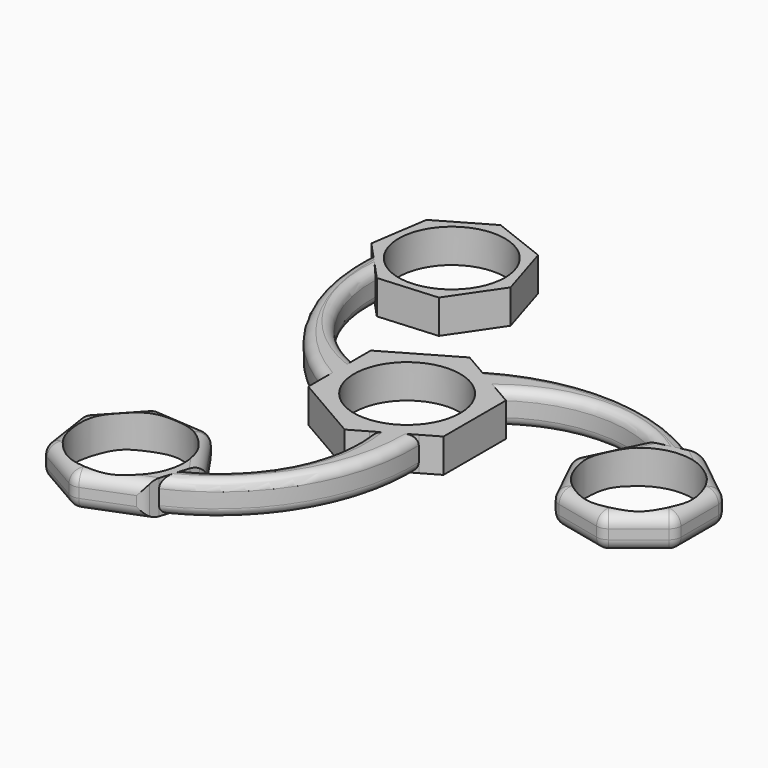
from build123d import *

# Parameters (mm, degrees)
F0_R          = 11
F1_DEPTH      = 7
F2_T4_ANGLE   = 80.8071756388
F2_T10_ANGLE  = 80.8071756388
F2_T16_ANGLE  = 89.7153399134
F2_T22_ANGLE  = 89.7153399134
F2_T28_ANGLE  = 80.8071756388
F2_T34_ANGLE  = 89.7153399134
F2_T40_ANGLE  = 80.8071756388
F2_T46_ANGLE  = 89.7153399134
F2_T52_ANGLE  = 89.7153399134
F2_T58_ANGLE  = 80.8071756388
F2_T64_ANGLE  = 89.7153399134
F2_T70_ANGLE  = 80.8071756388
F3_T1_DEPTH   = 9.7342520499
F3_T3_DEPTH   = 9.7342520499
F3_T5_DEPTH   = 9.7342520499
F3_T7_DEPTH   = 9.7342520499
F3_T9_DEPTH   = 17.188188597
F3_T11_DEPTH  = 2
F3_T13_DEPTH  = 13.0196827351
F3_T15_DEPTH  = 17.188188597
F3_T17_DEPTH  = 9.7342520499
F3_T19_DEPTH  = 9.7342520499
F3_T21_DEPTH  = 9.7342520499
F3_T23_DEPTH  = 9.7342520499
F3_T28_DEPTH  = 2.55
F3_T34_DEPTH  = 2.55
F3_T40_DEPTH  = 2.55
F3_T46_DEPTH  = 2.55
F3_T52_DEPTH  = 2.55
F3_T58_DEPTH  = 2.55
F3_T64_DEPTH  = 2.55
F3_T70_DEPTH  = 2.55
F3_T76_DEPTH  = 2.55
F3_T82_DEPTH  = 2.55
F3_T88_DEPTH  = 2.55
F3_T94_DEPTH  = 2.55
F3_T100_DEPTH = 2.55
F3_T106_DEPTH = 2.55
F3_T112_DEPTH = 2.55
F3_T118_DEPTH = 2.55
F3_T124_DEPTH = 2.55
F3_T130_DEPTH = 2.55
F3_T136_DEPTH = 2.55
F3_T142_DEPTH = 2.55
F3_T148_DEPTH = 17.188188597
F3_T153_DEPTH = 17.188188597
F3_T158_DEPTH = 17.188188597
F3_T163_DEPTH = 17.188188597


# Not quite as in the source:
# - a fillet or chamfer that OpenCascade refuses, or shapes differently, is made with other operations: its cross-section is extruded or revolved along the edge and cut away or added


with BuildPart() as f1:
    # F0 (on Top) → F1 (new body)
    with BuildSketch(Plane.XY):
        with BuildLine():
            Line((60.599063076, -6.071062572), (60.599063076, 6.071062572))
            Line((60.599063076, 6.071062572), (51.1059673744, 13.6415537722))
            Line((51.1059673744, 13.6415537722), (48.1465431954, 12.9660845153))
            ThreePointArc((48.1465431954, 12.9660845153), (25.9998304631, 20.2415563694), (3.5, 14.1450815951))
            Line((3.5, 14.1450815951), (0, 16.1658075373))
            Line((0, 16.1658075373), (-14, 8.0829037687))
            Line((-14, 8.0829037687), (-14, 4.0414518843))
            ThreePointArc((-14, 4.0414518843), (-26.7485538416, 14.727206882), (-31.1728589248, 30.7626834715))
            Line((-31.1728589248, 30.7626834715), (-29.1081732994, 28.5374815803))
            Line((-29.1081732994, 28.5374815803), (-17, 29.4448637287))
            Line((-17, 29.4448637287), (-10.1600973589, 39.4771583252))
            Line((-10.1600973589, 39.4771583252), (-13.7390515734, 51.0798429173))
            Line((-13.7390515734, 51.0798429173), (-25.0418371227, 55.5158593554))
            Line((-25.0418371227, 55.5158593554), (-35.5572259533, 49.4447967834))
            Line((-35.5572259533, 49.4447967834), (-37.366915801, 37.4382891451))
            Line((-37.366915801, 37.4382891451), (-35.3022301756, 35.2130872539))
            ThreePointArc((-35.3022301756, 35.2130872539), (-30.5296172596, 12.3957354905), (-14, -4.0414518843))
            Line((-14, -4.0414518843), (-14, -8.0829037687))
            Line((-14, -8.0829037687), (0, -16.1658075373))
            Line((0, -16.1658075373), (3.5, -14.1450815951))
            ThreePointArc((3.5, -14.1450815951), (0.6201416342, -30.5285305823), (-11.0548359125, -42.3778294732))
            Line((-11.0548359125, -42.3778294732), (-10.1600973589, -39.4771583252))
            Line((-10.1600973589, -39.4771583252), (-17, -29.4448637287))
            Line((-17, -29.4448637287), (-29.1081732994, -28.5374815803))
            Line((-29.1081732994, -28.5374815803), (-37.366915801, -37.4382891451))
            Line((-37.366915801, -37.4382891451), (-35.5572259533, -49.4447967834))
            Line((-35.5572259533, -49.4447967834), (-25.0418371227, -55.5158593554))
            Line((-25.0418371227, -55.5158593554), (-13.7390515734, -51.0798429173))
            Line((-13.7390515734, -51.0798429173), (-12.8443130198, -48.1791717693))
            ThreePointArc((-12.8443130198, -48.1791717693), (4.5297867965, -32.6372918599), (10.5, -10.1036297108))
            Line((10.5, -10.1036297108), (14, -8.0829037687))
            Line((14, -8.0829037687), (14, 0))
            Line((14, 0), (14, 8.0829037687))
            Line((14, 8.0829037687), (10.5, 10.1036297108))
            ThreePointArc((10.5, 10.1036297108), (26.1284122074, 15.8013237004), (42.2276948373, 11.6151460017))
            Line((42.2276948373, 11.6151460017), (39.2682706583, 10.9396767449))
            Line((39.2682706583, 10.9396767449), (34, 0))
            Line((34, 0), (39.2682706583, -10.9396767449))
            Line((39.2682706583, -10.9396767449), (51.1059673744, -13.6415537722))
            Line((51.1059673744, -13.6415537722), (60.599063076, -6.071062572))
        make_face()
        with Locations((-23.9961858727, -41.5626131193)):
            Circle(F0_R, mode=Mode.SUBTRACT)
        Circle(F0_R, mode=Mode.SUBTRACT)
        with Locations((47.9923717453, 0)):
            Circle(F0_R, mode=Mode.SUBTRACT)
        with Locations((-23.9961858727, 41.5626131193)):
            Circle(F0_R, mode=Mode.SUBTRACT)
    extrude(amount=F1_DEPTH)

    # F2: fillet of radius 2 on 12 edges, made by hand


with BuildPart() as f2_tool2:
    # F2_s3 → F2_t4 (revolve)
    with BuildSketch(Plane(origin=(6.6396058585, 31.4629160647, 0), x_dir=(0, 0, 1), z_dir=(0.2064819747, 0.9784504045, 0))):
        with BuildLine():
            ThreePointArc((7.0004, -40.1191282619), (6.4142135624, -41.5343075097), (4.9990343146, -42.1204939473))
            Line((4.9990343146, -42.1204939473), (4.9990343146, -42.3206305158))
            ThreePointArc((4.9990343146, -42.3206305158), (5.9995171573, -42.3202305158), (7, -42.3202305158))
            Line((7, -42.3202305158), (7.2001365685, -42.1200939473))
            ThreePointArc((7.2001365685, -42.1200939473), (7.2001365685, -41.1196111046), (7.2005365685, -40.1191282619))
            Line((7.2005365685, -40.1191282619), (7.0004, -40.1191282619))
        make_face()
    revolve(axis=Axis((5.1756088553, 31.7718627325, 7), (0, 0, 1)), revolution_arc=F2_T4_ANGLE)

    split(bisect_by=Plane.YZ.offset(-14), keep=Keep.BOTTOM)

    split(bisect_by=Plane(origin=(-1.4128724102, -1.310954016, 0), x_dir=(0, 0, 1), z_dir=(-0.7330518718, -0.6801727378, 0)), keep=Keep.TOP)


with BuildPart() as f1_1:
    add(f1.part)

    # F2_t1: cut F2_tool2
    add(f2_tool2.part, mode=Mode.SUBTRACT)


with BuildPart() as f2_tool8:
    # F2_s9 → F2_t10 (revolve)
    with BuildSketch(Plane(origin=(-30.5674875184, -9.9813906878, 0), x_dir=(0, 0, 1), z_dir=(-0.950603894, -0.3104065668, 0))):
        with BuildLine():
            ThreePointArc((7.0004, -40.1191282619), (6.4142135624, -41.5343075097), (4.9990343146, -42.1204939473))
            Line((4.9990343146, -42.1204939473), (4.9990343146, -42.3206305158))
            ThreePointArc((4.9990343146, -42.3206305158), (5.9995171573, -42.3202305158), (7, -42.3202305158))
            Line((7, -42.3202305158), (7.2001365685, -42.1200939473))
            ThreePointArc((7.2001365685, -42.1200939473), (7.2001365685, -41.1196111046), (7.2005365685, -40.1191282619))
            Line((7.2005365685, -40.1191282619), (7.0004, -40.1191282619))
        make_face()
    revolve(axis=Axis((-30.1030446796, -11.4037226175, 7), (0, 0, 1)), revolution_arc=F2_T10_ANGLE)

    split(bisect_by=Plane(origin=(7, -12.124355653, 0), x_dir=(0, 0, 1), z_dir=(0.5, -0.8660254038, 0)), keep=Keep.TOP)

    split(bisect_by=Plane(origin=(1.8417556862, -0.5681063915, 0), x_dir=(0, 0, 1), z_dir=(0.9555728058, -0.2947551744, 0)), keep=Keep.TOP)


with BuildPart() as f1_2:
    add(f1_1.part)

    # F2_t7: cut F2_tool8
    add(f2_tool8.part, mode=Mode.SUBTRACT)


with BuildPart() as f2_tool14:
    # F2_s15 → F2_t16 (revolve)
    with BuildSketch(Plane(origin=(2.8896760525, -9.1175868054, 0), x_dir=(0, 0, 1), z_dir=(-0.3021235761, 0.9532687684, 0))):
        with BuildLine():
            ThreePointArc((7.0004, 1.5102904536), (6.4142135624, 0.0951112058), (4.9990343146, -0.4910752318))
            Line((4.9990343146, -0.4910752318), (4.9990343146, -0.6912118004))
            ThreePointArc((4.9990343146, -0.6912118004), (5.9995171573, -0.6908118004), (7, -0.6908118004))
            Line((7, -0.6908118004), (7.2001365685, -0.4906752318))
            ThreePointArc((7.2001365685, -0.4906752318), (7.2001365685, 0.5098076109), (7.2005365685, 1.5102904536))
            Line((7.2005365685, 1.5102904536), (7.0004, 1.5102904536))
        make_face()
    revolve(axis=Axis((-24.2357516221, -17.714565418, 7), (0, 0, -1)), revolution_arc=F2_T16_ANGLE)

    split(bisect_by=Plane(origin=(1.8417556862, -0.5681063915, 0), x_dir=(0, 0, 1), z_dir=(0.9555728058, -0.2947551744, 0)), keep=Keep.TOP)

    split(bisect_by=Plane(origin=(7, -12.124355653, 0), x_dir=(0, 0, 1), z_dir=(0.5, -0.8660254038, 0)), keep=Keep.TOP)


with BuildPart() as f1_3:
    add(f1_2.part)

    # F2_t13: cut F2_tool14
    add(f2_tool14.part, mode=Mode.SUBTRACT)


with BuildPart() as f2_tool20:
    # F2_s21 → F2_t22 (revolve)
    with BuildSketch(Plane(origin=(6.4512237685, 7.0613262729, 0), x_dir=(0, 0, 1), z_dir=(-0.674493182, -0.7382810762, 0))):
        with BuildLine():
            ThreePointArc((7.0004, 1.5102904536), (6.4142135624, 0.0951112058), (4.9990343146, -0.4910752318))
            Line((4.9990343146, -0.4910752318), (4.9990343146, -0.6912118004))
            ThreePointArc((4.9990343146, -0.6912118004), (5.9995171573, -0.6908118004), (7, -0.6908118004))
            Line((7, -0.6908118004), (7.2001365685, -0.4906752318))
            ThreePointArc((7.2001365685, -0.4906752318), (7.2001365685, 0.5098076109), (7.2005365685, 1.5102904536))
            Line((7.2005365685, 1.5102904536), (7.0004, 1.5102904536))
        make_face()
    revolve(axis=Axis((27.45913948, -12.1314938756, 7), (0, 0, -1)), revolution_arc=F2_T22_ANGLE)

    split(bisect_by=Plane(origin=(-0.428883276, 1.8790604075, 0), x_dir=(0, 0, 1), z_dir=(-0.222520934, 0.9749279122, 0)), keep=Keep.TOP)

    split(bisect_by=Plane(origin=(7, 12.124355653, 0), x_dir=(0, 0, 1), z_dir=(0.5, 0.8660254038, 0)), keep=Keep.TOP)


with BuildPart() as f1_4:
    add(f1_3.part)

    # F2_t19: cut F2_tool20
    add(f2_tool20.part, mode=Mode.SUBTRACT)


with BuildPart() as f2_tool26:
    # F2_s27 → F2_t28 (revolve)
    with BuildSketch(Plane(origin=(23.9278816599, -21.4815253769, 0), x_dir=(0, 0, 1), z_dir=(0.7441219193, -0.6680438378, 0))):
        with BuildLine():
            ThreePointArc((7.0004, -40.1191282619), (6.4142135624, -41.5343075097), (4.9990343146, -42.1204939473))
            Line((4.9990343146, -42.1204939473), (4.9990343146, -42.3206305158))
            ThreePointArc((4.9990343146, -42.3206305158), (5.9995171573, -42.3202305158), (7, -42.3202305158))
            Line((7, -42.3202305158), (7.2001365685, -42.1200939473))
            ThreePointArc((7.2001365685, -42.1200939473), (7.2001365685, -41.1196111046), (7.2005365685, -40.1191282619))
            Line((7.2005365685, -40.1191282619), (7.0004, -40.1191282619))
        make_face()
    revolve(axis=Axis((24.9274358243, -20.368140115, 7), (0, 0, 1)), revolution_arc=F2_T28_ANGLE)

    split(bisect_by=Plane(origin=(7, 12.124355653, 0), x_dir=(0, 0, 1), z_dir=(0.5, 0.8660254038, 0)), keep=Keep.TOP)

    split(bisect_by=Plane(origin=(-0.428883276, 1.8790604075, 0), x_dir=(0, 0, 1), z_dir=(-0.222520934, 0.9749279122, 0)), keep=Keep.TOP)


with BuildPart() as f1_5:
    add(f1_4.part)

    # F2_t25: cut F2_tool26
    add(f2_tool26.part, mode=Mode.SUBTRACT)


with BuildPart() as f2_tool32:
    # F2_s33 → F2_t34 (revolve)
    with BuildSketch(Plane(origin=(-9.3408998209, 2.0562605326, 0), x_dir=(0, 0, 1), z_dir=(0.9766167581, -0.2149876922, 0))):
        with BuildLine():
            ThreePointArc((7.0004, 1.5102904536), (6.4142135624, 0.0951112058), (4.9990343146, -0.4910752318))
            Line((4.9990343146, -0.4910752318), (4.9990343146, -0.6912118004))
            ThreePointArc((4.9990343146, -0.6912118004), (5.9995171573, -0.6908118004), (7, -0.6908118004))
            Line((7, -0.6908118004), (7.2001365685, -0.4906752318))
            ThreePointArc((7.2001365685, -0.4906752318), (7.2001365685, 0.5098076109), (7.2005365685, 1.5102904536))
            Line((7.2005365685, 1.5102904536), (7.0004, 1.5102904536))
        make_face()
    revolve(axis=Axis((-3.2233878579, 29.8460592935, 7), (0, 0, -1)), revolution_arc=F2_T34_ANGLE)

    split(bisect_by=Plane(origin=(-1.4128724102, -1.310954016, 0), x_dir=(0, 0, 1), z_dir=(-0.7330518718, -0.6801727378, 0)), keep=Keep.TOP)

    split(bisect_by=Plane.YZ.offset(-14), keep=Keep.BOTTOM)


with BuildPart() as f1_6:
    add(f1_5.part)

    # F2_t31: cut F2_tool32
    add(f2_tool32.part, mode=Mode.SUBTRACT)


with BuildPart() as f2_tool38:
    # F2_s39 → F2_t40 (revolve)
    with BuildSketch(Plane(origin=(-30.5674875184, -9.9813906878, 0), x_dir=(0, 0, 1), z_dir=(-0.950603894, -0.3104065668, 0))):
        with BuildLine():
            ThreePointArc((2.0009656854, -42.1204939473), (0.5857864376, -41.5343075097), (-0.0004, -40.1191282619))
            Line((-0.0004, -40.1191282619), (-0.2005365685, -40.1191282619))
            ThreePointArc((-0.2005365685, -40.1191282619), (-0.2001365685, -41.1196111046), (-0.2001365685, -42.1200939473))
            Line((-0.2001365685, -42.1200939473), (0, -42.3202305158))
            ThreePointArc((0, -42.3202305158), (1.0004828427, -42.3202305158), (2.0009656854, -42.3206305158))
            Line((2.0009656854, -42.3206305158), (2.0009656854, -42.1204939473))
        make_face()
    revolve(axis=Axis((-30.1030446796, -11.4037226175, 0), (0, 0, 1)), revolution_arc=F2_T40_ANGLE)

    split(bisect_by=Plane(origin=(7, -12.124355653, 0), x_dir=(0, 0, 1), z_dir=(0.5, -0.8660254038, 0)), keep=Keep.TOP)

    split(bisect_by=Plane(origin=(1.8417556862, -0.5681063915, 0), x_dir=(0, 0, 1), z_dir=(0.9555728058, -0.2947551744, 0)), keep=Keep.TOP)


with BuildPart() as f1_7:
    add(f1_6.part)

    # F2_t37: cut F2_tool38
    add(f2_tool38.part, mode=Mode.SUBTRACT)


with BuildPart() as f2_tool44:
    # F2_s45 → F2_t46 (revolve)
    with BuildSketch(Plane(origin=(2.8896760525, -9.1175868054, 0), x_dir=(0, 0, 1), z_dir=(-0.3021235761, 0.9532687684, 0))):
        with BuildLine():
            ThreePointArc((2.0009656854, -0.4910752318), (0.5857864376, 0.0951112058), (-0.0004, 1.5102904536))
            Line((-0.0004, 1.5102904536), (-0.2005365685, 1.5102904536))
            ThreePointArc((-0.2005365685, 1.5102904536), (-0.2001365685, 0.5098076109), (-0.2001365685, -0.4906752318))
            Line((-0.2001365685, -0.4906752318), (0, -0.6908118004))
            ThreePointArc((0, -0.6908118004), (1.0004828427, -0.6908118004), (2.0009656854, -0.6912118004))
            Line((2.0009656854, -0.6912118004), (2.0009656854, -0.4910752318))
        make_face()
    revolve(axis=Axis((-24.2357516221, -17.714565418, 0), (0, 0, -1)), revolution_arc=F2_T46_ANGLE)

    split(bisect_by=Plane(origin=(1.8417556862, -0.5681063915, 0), x_dir=(0, 0, 1), z_dir=(0.9555728058, -0.2947551744, 0)), keep=Keep.TOP)

    split(bisect_by=Plane(origin=(7, -12.124355653, 0), x_dir=(0, 0, 1), z_dir=(0.5, -0.8660254038, 0)), keep=Keep.TOP)


with BuildPart() as f1_8:
    add(f1_7.part)

    # F2_t43: cut F2_tool44
    add(f2_tool44.part, mode=Mode.SUBTRACT)


with BuildPart() as f2_tool50:
    # F2_s51 → F2_t52 (revolve)
    with BuildSketch(Plane(origin=(6.4512237685, 7.0613262729, 0), x_dir=(0, 0, 1), z_dir=(-0.674493182, -0.7382810762, 0))):
        with BuildLine():
            ThreePointArc((2.0009656854, -0.4910752318), (0.5857864376, 0.0951112058), (-0.0004, 1.5102904536))
            Line((-0.0004, 1.5102904536), (-0.2005365685, 1.5102904536))
            ThreePointArc((-0.2005365685, 1.5102904536), (-0.2001365685, 0.5098076109), (-0.2001365685, -0.4906752318))
            Line((-0.2001365685, -0.4906752318), (0, -0.6908118004))
            ThreePointArc((0, -0.6908118004), (1.0004828427, -0.6908118004), (2.0009656854, -0.6912118004))
            Line((2.0009656854, -0.6912118004), (2.0009656854, -0.4910752318))
        make_face()
    revolve(axis=Axis((27.45913948, -12.1314938756, 0), (0, 0, -1)), revolution_arc=F2_T52_ANGLE)

    split(bisect_by=Plane(origin=(-0.428883276, 1.8790604075, 0), x_dir=(0, 0, 1), z_dir=(-0.222520934, 0.9749279122, 0)), keep=Keep.TOP)

    split(bisect_by=Plane(origin=(7, 12.124355653, 0), x_dir=(0, 0, 1), z_dir=(0.5, 0.8660254038, 0)), keep=Keep.TOP)


with BuildPart() as f1_9:
    add(f1_8.part)

    # F2_t49: cut F2_tool50
    add(f2_tool50.part, mode=Mode.SUBTRACT)


with BuildPart() as f2_tool56:
    # F2_s57 → F2_t58 (revolve)
    with BuildSketch(Plane(origin=(23.9278816599, -21.4815253769, 0), x_dir=(0, 0, 1), z_dir=(0.7441219193, -0.6680438378, 0))):
        with BuildLine():
            ThreePointArc((2.0009656854, -42.1204939473), (0.5857864376, -41.5343075097), (-0.0004, -40.1191282619))
            Line((-0.0004, -40.1191282619), (-0.2005365685, -40.1191282619))
            ThreePointArc((-0.2005365685, -40.1191282619), (-0.2001365685, -41.1196111046), (-0.2001365685, -42.1200939473))
            Line((-0.2001365685, -42.1200939473), (0, -42.3202305158))
            ThreePointArc((0, -42.3202305158), (1.0004828427, -42.3202305158), (2.0009656854, -42.3206305158))
            Line((2.0009656854, -42.3206305158), (2.0009656854, -42.1204939473))
        make_face()
    revolve(axis=Axis((24.9274358243, -20.368140115, 0), (0, 0, 1)), revolution_arc=F2_T58_ANGLE)

    split(bisect_by=Plane(origin=(7, 12.124355653, 0), x_dir=(0, 0, 1), z_dir=(0.5, 0.8660254038, 0)), keep=Keep.TOP)

    split(bisect_by=Plane(origin=(-0.428883276, 1.8790604075, 0), x_dir=(0, 0, 1), z_dir=(-0.222520934, 0.9749279122, 0)), keep=Keep.TOP)


with BuildPart() as f1_10:
    add(f1_9.part)

    # F2_t55: cut F2_tool56
    add(f2_tool56.part, mode=Mode.SUBTRACT)


with BuildPart() as f2_tool62:
    # F2_s63 → F2_t64 (revolve)
    with BuildSketch(Plane(origin=(-9.3408998209, 2.0562605326, 0), x_dir=(0, 0, 1), z_dir=(0.9766167581, -0.2149876922, 0))):
        with BuildLine():
            ThreePointArc((2.0009656854, -0.4910752318), (0.5857864376, 0.0951112058), (-0.0004, 1.5102904536))
            Line((-0.0004, 1.5102904536), (-0.2005365685, 1.5102904536))
            ThreePointArc((-0.2005365685, 1.5102904536), (-0.2001365685, 0.5098076109), (-0.2001365685, -0.4906752318))
            Line((-0.2001365685, -0.4906752318), (0, -0.6908118004))
            ThreePointArc((0, -0.6908118004), (1.0004828427, -0.6908118004), (2.0009656854, -0.6912118004))
            Line((2.0009656854, -0.6912118004), (2.0009656854, -0.4910752318))
        make_face()
    revolve(axis=Axis((-3.2233878579, 29.8460592935, 0), (0, 0, -1)), revolution_arc=F2_T64_ANGLE)

    split(bisect_by=Plane(origin=(-1.4128724102, -1.310954016, 0), x_dir=(0, 0, 1), z_dir=(-0.7330518718, -0.6801727378, 0)), keep=Keep.TOP)

    split(bisect_by=Plane.YZ.offset(-14), keep=Keep.BOTTOM)


with BuildPart() as f1_11:
    add(f1_10.part)

    # F2_t61: cut F2_tool62
    add(f2_tool62.part, mode=Mode.SUBTRACT)


with BuildPart() as f2_tool68:
    # F2_s69 → F2_t70 (revolve)
    with BuildSketch(Plane(origin=(6.6396058585, 31.4629160647, 0), x_dir=(0, 0, 1), z_dir=(0.2064819747, 0.9784504045, 0))):
        with BuildLine():
            ThreePointArc((2.0009656854, -42.1204939473), (0.5857864376, -41.5343075097), (-0.0004, -40.1191282619))
            Line((-0.0004, -40.1191282619), (-0.2005365685, -40.1191282619))
            ThreePointArc((-0.2005365685, -40.1191282619), (-0.2001365685, -41.1196111046), (-0.2001365685, -42.1200939473))
            Line((-0.2001365685, -42.1200939473), (0, -42.3202305158))
            ThreePointArc((0, -42.3202305158), (1.0004828427, -42.3202305158), (2.0009656854, -42.3206305158))
            Line((2.0009656854, -42.3206305158), (2.0009656854, -42.1204939473))
        make_face()
    revolve(axis=Axis((5.1756088553, 31.7718627325, 0), (0, 0, 1)), revolution_arc=F2_T70_ANGLE)

    split(bisect_by=Plane.YZ.offset(-14), keep=Keep.BOTTOM)

    split(bisect_by=Plane(origin=(-1.4128724102, -1.310954016, 0), x_dir=(0, 0, 1), z_dir=(-0.7330518718, -0.6801727378, 0)), keep=Keep.TOP)


with BuildPart() as f1_12:
    add(f1_11.part)

    # F2_t67: cut F2_tool68
    add(f2_tool68.part, mode=Mode.SUBTRACT)

    # F3: fillet of radius 2.5 on 38 edges, made by hand

    # F3_s2 → F3_t1 (cut)
    with BuildSketch(Plane(origin=(-28.5141857065, -30.7309835357, 0), x_dir=(0, 0, 1), z_dir=(-0.6801727378, -0.7330518718, 0))):
        with BuildLine():
            ThreePointArc((2.5, 1.9273839471), (0.732233047, 1.1951509001), (0, -0.5726160529))
            Line((0, -0.5726160529), (0, 1.9273839471))
            Line((0, 1.9273839471), (2.5, 1.9273839471))
        make_face()
        with BuildLine():
            ThreePointArc((4.5, 1.9273839471), (6.267766953, 1.1951509001), (7, -0.5726160529))
            Line((7, -0.5726160529), (7, 1.9273839471))
            Line((7, 1.9273839471), (4.5, 1.9273839471))
        make_face()
    extrude(amount=F3_T1_DEPTH, mode=Mode.SUBTRACT)

    # F3_s4 → F3_t3 (cut)
    with BuildSketch(Plane(origin=(4.8669485419, -32.2900937521, 0), x_dir=(0, 0, 1), z_dir=(0.1490422662, -0.9888308262, 0))):
        with BuildLine():
            ThreePointArc((0, 40.0294456809), (0.732233047, 41.7972126339), (2.5, 42.5294456809))
            Line((2.5, 42.5294456809), (0, 42.5294456809))
            Line((0, 42.5294456809), (0, 40.0294456809))
        make_face()
        with BuildLine():
            ThreePointArc((7, 40.0294456809), (6.267766953, 41.7972126339), (4.5, 42.5294456809))
            Line((4.5, 42.5294456809), (7, 42.5294456809))
            Line((7, 42.5294456809), (7, 40.0294456809))
        make_face()
    extrude(amount=F3_T3_DEPTH, mode=Mode.SUBTRACT)

    # F3_s6 → F3_t5 (cut)
    with BuildSketch(Plane(origin=(-4.215054781, 2.4335630125, 0), x_dir=(0, 0, 1), z_dir=(0.8660254038, -0.5, 0))):
        with BuildLine():
            ThreePointArc((2.5, 60.599063076), (0.732233047, 59.866830029), (0, 58.099063076))
            Line((0, 58.099063076), (0, 60.599063076))
            Line((0, 60.599063076), (2.5, 60.599063076))
        make_face()
        with BuildLine():
            ThreePointArc((7, 58.099063076), (6.267766953, 59.866830029), (4.5, 60.599063076))
            Line((4.5, 60.599063076), (7, 60.599063076))
            Line((7, 60.599063076), (7, 58.099063076))
        make_face()
    extrude(amount=F3_T5_DEPTH, mode=Mode.SUBTRACT)

    # F3_s8 → F3_t7 (cut)
    with BuildSketch(Plane(origin=(-15.9113675105, 1.1923921534, 0), x_dir=(0, 0, 1), z_dir=(-0.9972037972, 0.0747300936, 0))):
        with BuildLine():
            ThreePointArc((0, -33.1329415087), (0.732233047, -31.3651745557), (2.5, -30.6329415087))
            Line((2.5, -30.6329415087), (0, -30.6329415087))
            Line((0, -30.6329415087), (0, -33.1329415087))
        make_face()
        with BuildLine():
            ThreePointArc((7, -33.1329415087), (6.267766953, -31.3651745557), (4.5, -30.6329415087))
            Line((4.5, -30.6329415087), (7, -30.6329415087))
            Line((7, -30.6329415087), (7, -33.1329415087))
        make_face()
    extrude(amount=F3_T7_DEPTH, mode=Mode.SUBTRACT)

    # F3_s10 → F3_t9 (cut)
    with BuildSketch(Plane(origin=(-39.4588754468, -15.4864674153, 0), x_dir=(0, 0, 1), z_dir=(0.9308737486, 0.3653410244, 0))):
        with BuildLine():
            ThreePointArc((2.5, 42.5294456809), (0.732233047, 41.7972126339), (0, 40.0294456809))
            Line((0, 40.0294456809), (0, 42.5294456809))
            Line((0, 42.5294456809), (2.5, 42.5294456809))
        make_face()
        with BuildLine():
            ThreePointArc((7, 40.0294456809), (6.267766953, 41.7972126339), (4.5, 42.5294456809))
            Line((4.5, 42.5294456809), (7, 42.5294456809))
            Line((7, 42.5294456809), (7, 40.0294456809))
        make_face()
    extrude(amount=F3_T9_DEPTH, mode=Mode.SUBTRACT)

    # F3_s12 → F3_t11 (cut)
    with BuildSketch(Plane.XY.offset(2.5)):
        with BuildLine():
            ThreePointArc((-36.5480309837, -36.5557412058), (-37.1043333186, -37.5192851142), (-37.1874783697, -38.6287787156))
            Line((-37.1874783697, -38.6287787156), (-37.366915801, -37.4382891451))
            Line((-37.366915801, -37.4382891451), (-36.5480309837, -36.5557412058))
        make_face()
        with BuildLine():
            ThreePointArc((-34.5145863191, -50.0467650569), (-35.3301832548, -49.2900016926), (-35.7366633846, -48.2543072129))
            Line((-35.7366633846, -48.2543072129), (-35.5572259533, -49.4447967834))
            Line((-35.5572259533, -49.4447967834), (-34.5145863191, -50.0467650569))
        make_face()
        with BuildLine():
            ThreePointArc((-23.921124196, -55.076011944), (-25.0213019909, -55.2418370653), (-26.084476757, -54.9138910819))
            Line((-26.084476757, -54.9138910819), (-25.0418371227, -55.5158593554))
            Line((-25.0418371227, -55.5158593554), (-23.921124196, -55.076011944))
        make_face()
        with BuildLine():
            ThreePointArc((-29.9270581167, -29.4200295197), (-29.0077809981, -28.7932769925), (-27.9076032032, -28.6274518712))
            Line((-27.9076032032, -28.6274518712), (-29.1081732994, -28.5374815803))
            Line((-29.1081732994, -28.5374815803), (-29.9270581167, -29.4200295197))
        make_face()
        with BuildLine():
            ThreePointArc((-16.3217983944, -30.4396027856), (-17.1373953302, -29.6828394213), (-18.2005700963, -29.3548934378))
            Line((-18.2005700963, -29.3548934378), (-17, -29.4448637287))
            Line((-17, -29.4448637287), (-16.3217983944, -30.4396027856))
        make_face()
        with BuildLine():
            ThreePointArc((59.6577875807, 6.8217047311), (60.3514852458, 5.9518353728), (60.599063076, 4.867126025))
            Line((60.599063076, 4.867126025), (60.599063076, 6.071062572))
            Line((60.599063076, 6.071062572), (59.6577875807, 6.8217047311))
        make_face()
        with BuildLine():
            ThreePointArc((60.599063076, -4.867126025), (60.3514852458, -5.9518353728), (59.6577875807, -6.8217047311))
            Line((59.6577875807, -6.8217047311), (60.599063076, -6.071062572))
            Line((60.599063076, -6.071062572), (60.599063076, -4.867126025))
        make_face()
        with BuildLine():
            ThreePointArc((52.0472428697, -12.890911613), (51.0448207, -13.3736526873), (49.9322160302, -13.3736526873))
            Line((49.9322160302, -13.3736526873), (51.1059673744, -13.6415537722))
            Line((51.1059673744, -13.6415537722), (52.0472428697, -12.890911613))
        make_face()
        with BuildLine():
            ThreePointArc((40.4420220025, -11.2075778298), (39.4395998327, -10.7248367555), (38.7459021676, -9.8549673971))
            Line((38.7459021676, -9.8549673971), (39.2682706583, -10.9396767449))
            Line((39.2682706583, -10.9396767449), (40.4420220025, -11.2075778298))
        make_face()
        with BuildLine():
            ThreePointArc((34.5223684907, -1.0847093478), (34.2747906604, 0), (34.5223684907, 1.0847093478))
            Line((34.5223684907, 1.0847093478), (34, 0))
            Line((34, 0), (34.5223684907, -1.0847093478))
        make_face()
    extrude(amount=F3_T11_DEPTH, mode=Mode.SUBTRACT)

    # F3_s14 → F3_t13 (cut)
    with BuildSketch(Plane.XY.offset(-3.0098413675)):
        with BuildLine():
            ThreePointArc((-10.8382989644, -38.4824192683), (-10.4318188347, -39.518113748), (-10.5149638858, -40.6276073495))
            Line((-10.5149638858, -40.6276073495), (-10.1600973589, -39.4771583252))
            Line((-10.1600973589, -39.4771583252), (-10.8382989644, -38.4824192683))
        make_face()
        with BuildLine():
            ThreePointArc((-13.3841850465, -49.929393893), (-13.9404873814, -50.8929378014), (-14.8597645001, -51.5196903286))
            Line((-14.8597645001, -51.5196903286), (-13.7390515734, -51.0798429173))
            Line((-13.7390515734, -51.0798429173), (-13.3841850465, -49.929393893))
        make_face()
        with BuildLine():
            ThreePointArc((49.9322160302, 13.3736526873), (51.0448207, 13.3736526873), (52.0472428697, 12.890911613))
            Line((52.0472428697, 12.890911613), (51.1059673744, 13.6415537722))
            Line((51.1059673744, 13.6415537722), (49.9322160302, 13.3736526873))
        make_face()
        with BuildLine():
            ThreePointArc((38.7459021676, 9.8549673971), (39.4395998327, 10.7248367555), (40.4420220025, 11.2075778298))
            Line((40.4420220025, 11.2075778298), (39.2682706583, 10.9396767449))
            Line((39.2682706583, 10.9396767449), (38.7459021676, 9.8549673971))
        make_face()
    extrude(amount=F3_T13_DEPTH, mode=Mode.SUBTRACT)

    # F3_s16 → F3_t15 (cut)
    with BuildSketch(Plane(origin=(33.1411119199, -26.4291548341, 0), x_dir=(0, 0, 1), z_dir=(-0.7818314825, 0.6234898019, 0))):
        with BuildLine():
            ThreePointArc((2.5, 42.5294456809), (0.732233047, 41.7972126339), (0, 40.0294456809))
            Line((0, 40.0294456809), (0, 42.5294456809))
            Line((0, 42.5294456809), (2.5, 42.5294456809))
        make_face()
        with BuildLine():
            ThreePointArc((7, 40.0294456809), (6.267766953, 41.7972126339), (4.5, 42.5294456809))
            Line((4.5, 42.5294456809), (7, 42.5294456809))
            Line((7, 42.5294456809), (7, 40.0294456809))
        make_face()
    extrude(amount=F3_T15_DEPTH, mode=Mode.SUBTRACT)

    # F3_s18 → F3_t17 (cut)
    with BuildSketch(Plane.XZ.offset(-4.867126025)):
        with BuildLine():
            ThreePointArc((60.599063076, 2.5), (59.866830029, 0.732233047), (58.099063076, 0))
            Line((58.099063076, 0), (60.599063076, 0))
            Line((60.599063076, 0), (60.599063076, 2.5))
        make_face()
        with BuildLine():
            ThreePointArc((58.099063076, 7), (59.866830029, 6.267766953), (60.599063076, 4.5))
            Line((60.599063076, 4.5), (60.599063076, 7))
            Line((60.599063076, 7), (58.099063076, 7))
        make_face()
    extrude(amount=F3_T17_DEPTH, mode=Mode.SUBTRACT)

    # F3_s20 → F3_t19 (cut)
    with BuildSketch(Plane(origin=(25.530567209, 20.3599479522, 0), x_dir=(0, 0, 1), z_dir=(0.7818314825, 0.6234898019, 0))):
        with BuildLine():
            ThreePointArc((2.5, 42.5294456809), (0.732233047, 41.7972126339), (0, 40.0294456809))
            Line((0, 40.0294456809), (0, 42.5294456809))
            Line((0, 42.5294456809), (2.5, 42.5294456809))
        make_face()
        with BuildLine():
            ThreePointArc((7, 40.0294456809), (6.267766953, 41.7972126339), (4.5, 42.5294456809))
            Line((4.5, 42.5294456809), (7, 42.5294456809))
            Line((7, 42.5294456809), (7, 40.0294456809))
        make_face()
    extrude(amount=F3_T19_DEPTH, mode=Mode.SUBTRACT)

    # F3_s22 → F3_t21 (cut)
    with BuildSketch(Plane(origin=(40.8709052785, -9.3285174222, 0), x_dir=(0, 0, 1), z_dir=(0.9749279122, -0.222520934, 0))):
        with BuildLine():
            ThreePointArc((2.5, 1.9273839471), (0.732233047, 1.1951509001), (0, -0.5726160529))
            Line((0, -0.5726160529), (0, 1.9273839471))
            Line((0, 1.9273839471), (2.5, 1.9273839471))
        make_face()
        with BuildLine():
            ThreePointArc((7, -0.5726160529), (6.267766953, 1.1951509001), (4.5, 1.9273839471))
            Line((4.5, 1.9273839471), (7, 1.9273839471))
            Line((7, 1.9273839471), (7, -0.5726160529))
        make_face()
    extrude(amount=F3_T21_DEPTH, mode=Mode.SUBTRACT)

    # F3_s24 → F3_t23 (cut)
    with BuildSketch(Plane(origin=(6.9230418591, -14.3758445498, 0), x_dir=(0, 0, 1), z_dir=(0.4338837391, -0.9009688679, 0))):
        with BuildLine():
            ThreePointArc((2.5, -30.6329415087), (0.732233047, -31.3651745557), (0, -33.1329415087))
            Line((0, -33.1329415087), (0, -30.6329415087))
            Line((0, -30.6329415087), (2.5, -30.6329415087))
        make_face()
        with BuildLine():
            ThreePointArc((7, -33.1329415087), (6.267766953, -31.3651745557), (4.5, -30.6329415087))
            Line((4.5, -30.6329415087), (7, -30.6329415087))
            Line((7, -30.6329415087), (7, -33.1329415087))
        make_face()
    extrude(amount=F3_T23_DEPTH, mode=Mode.SUBTRACT)


with BuildPart() as f3_tool26:
    # F3_s27 → F3_t28 (new body)
    with BuildSketch(Plane.XY.offset(2.5)):
        Polygon((-28.0944284371, -31.1204613641), (-29.9637107103, -29.3860208828), (-29.1284481967, -28.4858219846), (-27.9038666985, -28.5775916813), align=None)
    extrude(amount=-F3_T28_DEPTH)

    # F3_s29 → F3_t30 (revolve, cut)
    with BuildSketch(Plane(origin=(-28.0944284371, -31.1204613641, 2.5), x_dir=(0.3653410244, -0.9308737486, 0), z_dir=(0.9308737486, 0.3653410244, 0))):
        with BuildLine():
            ThreePointArc((0, -2.5), (2.5, 0), (0, 2.5))
            Line((0, 2.5), (0, -2.5))
        make_face()
    revolve(axis=Axis((-28.0944284371, -31.1204613641, 2.5), (0, 0, -1)), mode=Mode.SUBTRACT)


with BuildPart() as f1_13:
    add(f1_12.part)

    # F3_t25: cut F3_tool26
    add(f3_tool26.part, mode=Mode.SUBTRACT)


with BuildPart() as f3_tool32:
    # F3_s33 → F3_t34 (new body)
    with BuildSketch(Plane.XY.offset(2.5)):
        Polygon((-34.7154013041, -38.2561730502), (-37.236919911, -38.6362308289), (-37.4199460909, -37.421931467), (-36.5846835773, -36.5217325689), align=None)
    extrude(amount=-F3_T34_DEPTH)

    # F3_s35 → F3_t36 (revolve, cut)
    with BuildSketch(Plane(origin=(-34.7154013041, -38.2561730502, 2.5), x_dir=(0.9555728058, -0.2947551744, 0), z_dir=(0.2947551744, 0.9555728058, 0))):
        with BuildLine():
            ThreePointArc((0, -2.5), (2.5, 0), (0, 2.5))
            Line((0, 2.5), (0, -2.5))
        make_face()
    revolve(axis=Axis((-34.7154013041, -38.2561730502, 2.5), (0, 0, -1)), mode=Mode.SUBTRACT)


with BuildPart() as f1_14:
    add(f1_13.part)

    # F3_t31: cut F3_tool32
    add(f3_tool32.part, mode=Mode.SUBTRACT)


with BuildPart() as f3_tool38:
    # F3_s39 → F3_t40 (new body)
    with BuildSketch(Plane.XY.offset(2.5)):
        Polygon((-33.2645863191, -47.8817015474), (-35.7861049259, -48.2617593262), (-35.603078746, -49.4760586881), (-34.5395863191, -50.0900663271), align=None)
    extrude(amount=-F3_T40_DEPTH)

    # F3_s41 → F3_t42 (revolve, cut)
    with BuildSketch(Plane(origin=(-33.2645863191, -47.8817015474, 2.5), x_dir=(0.8262387743, 0.5633200581, 0), z_dir=(-0.5633200581, 0.8262387743, 0))):
        with BuildLine():
            ThreePointArc((0, -2.5), (2.5, 0), (0, 2.5))
            Line((0, 2.5), (0, -2.5))
        make_face()
    revolve(axis=Axis((-33.2645863191, -47.8817015474, 2.5), (0, 0, -1)), mode=Mode.SUBTRACT)


with BuildPart() as f1_15:
    add(f1_14.part)

    # F3_t37: cut F3_tool38
    add(f3_tool38.part, mode=Mode.SUBTRACT)


with BuildPart() as f3_tool44:
    # F3_s45 → F3_t46 (new body)
    with BuildSketch(Plane.XY.offset(2.5)):
        Polygon((-24.834476757, -52.7488275724), (-23.9028571448, -55.1225556314), (-25.04598433, -55.571199991), (-26.109476757, -54.957192352), align=None)
    extrude(amount=-F3_T46_DEPTH)

    # F3_s47 → F3_t48 (revolve, cut)
    with BuildSketch(Plane(origin=(-24.834476757, -52.7488275724, 2.5), x_dir=(0.0747300936, 0.9972037972, 0), z_dir=(-0.9972037972, 0.0747300936, 0))):
        with BuildLine():
            ThreePointArc((0, -2.5), (2.5, 0), (0, 2.5))
            Line((0, 2.5), (0, -2.5))
        make_face()
    revolve(axis=Axis((-24.834476757, -52.7488275724, 2.5), (0, 0, -1)), mode=Mode.SUBTRACT)


with BuildPart() as f1_16:
    add(f1_15.part)

    # F3_t43: cut F3_tool44
    add(f3_tool44.part, mode=Mode.SUBTRACT)


with BuildPart() as f3_tool50:
    # F3_s51 → F3_t52 (new body)
    with BuildSketch(Plane.XY.offset(2.5)):
        Polygon((-18.3873953302, -31.8479029308), (-18.1968335916, -29.305033248), (-16.9722520934, -29.3968029446), (-16.2804864557, -30.4114367827), align=None)
    extrude(amount=-F3_T52_DEPTH)

    # F3_s53 → F3_t54 (revolve, cut)
    with BuildSketch(Plane(origin=(-18.3873953302, -31.8479029308, 2.5), x_dir=(-0.5, -0.8660254038, 0), z_dir=(0.8660254038, -0.5, 0))):
        with BuildLine():
            ThreePointArc((0, -2.5), (2.5, 0), (0, 2.5))
            Line((0, 2.5), (0, -2.5))
        make_face()
    revolve(axis=Axis((-18.3873953302, -31.8479029308, 2.5), (0, 0, -1)), mode=Mode.SUBTRACT)


with BuildPart() as f1_17:
    add(f1_16.part)

    # F3_t49: cut F3_tool50
    add(f3_tool50.part, mode=Mode.SUBTRACT)


with BuildPart() as f3_tool56:
    # F3_s57 → F3_t58 (new body)
    with BuildSketch(Plane.XY.offset(4.5)):
        Polygon((-33.2645863191, -47.8817015474), (-34.5395863191, -50.0900663271), (-35.603078746, -49.4760586881), (-35.7861049259, -48.2617593262), align=None)
    extrude(amount=F3_T58_DEPTH)

    # F3_s59 → F3_t60 (revolve, cut)
    with BuildSketch(Plane(origin=(-33.2645863191, -47.8817015474, 4.5), x_dir=(0.8262387743, 0.5633200581, 0), z_dir=(0.5633200581, -0.8262387743, 0))):
        with BuildLine():
            ThreePointArc((0, -2.5), (2.5, 0), (0, 2.5))
            Line((0, 2.5), (0, -2.5))
        make_face()
    revolve(axis=Axis((-33.2645863191, -47.8817015474, 4.5), (0, 0, 1)), mode=Mode.SUBTRACT)


with BuildPart() as f1_18:
    add(f1_17.part)

    # F3_t55: cut F3_tool56
    add(f3_tool56.part, mode=Mode.SUBTRACT)


with BuildPart() as f3_tool62:
    # F3_s63 → F3_t64 (new body)
    with BuildSketch(Plane.XY.offset(4.5)):
        Polygon((-24.834476757, -52.7488275724), (-26.109476757, -54.957192352), (-25.04598433, -55.571199991), (-23.9028571448, -55.1225556314), align=None)
    extrude(amount=F3_T64_DEPTH)

    # F3_s65 → F3_t66 (revolve, cut)
    with BuildSketch(Plane(origin=(-24.834476757, -52.7488275724, 4.5), x_dir=(0.0747300936, 0.9972037972, 0), z_dir=(0.9972037972, -0.0747300936, 0))):
        with BuildLine():
            ThreePointArc((0, -2.5), (2.5, 0), (0, 2.5))
            Line((0, 2.5), (0, -2.5))
        make_face()
    revolve(axis=Axis((-24.834476757, -52.7488275724, 4.5), (0, 0, 1)), mode=Mode.SUBTRACT)


with BuildPart() as f1_19:
    add(f1_18.part)

    # F3_t61: cut F3_tool62
    add(f3_tool62.part, mode=Mode.SUBTRACT)


with BuildPart() as f3_tool68:
    # F3_s69 → F3_t70 (new body)
    with BuildSketch(Plane.XY.offset(4.5)):
        Polygon((-18.3873953302, -31.8479029308), (-16.2804864557, -30.4114367827), (-16.9722520934, -29.3968029446), (-18.1968335916, -29.305033248), align=None)
    extrude(amount=F3_T70_DEPTH)

    # F3_s71 → F3_t72 (revolve, cut)
    with BuildSketch(Plane(origin=(-18.3873953302, -31.8479029308, 4.5), x_dir=(-0.5, -0.8660254038, 0), z_dir=(-0.8660254038, 0.5, 0))):
        with BuildLine():
            ThreePointArc((0, -2.5), (2.5, 0), (0, 2.5))
            Line((0, 2.5), (0, -2.5))
        make_face()
    revolve(axis=Axis((-18.3873953302, -31.8479029308, 4.5), (0, 0, 1)), mode=Mode.SUBTRACT)


with BuildPart() as f1_20:
    add(f1_19.part)

    # F3_t67: cut F3_tool68
    add(f3_tool68.part, mode=Mode.SUBTRACT)


with BuildPart() as f3_tool74:
    # F3_s75 → F3_t76 (new body)
    with BuildSketch(Plane.XY.offset(4.5)):
        Polygon((-28.0944284371, -31.1204613641), (-29.9637107103, -29.3860208828), (-29.1284481967, -28.4858219846), (-27.9038666985, -28.5775916813), align=None)
    extrude(amount=F3_T76_DEPTH)

    # F3_s77 → F3_t78 (revolve, cut)
    with BuildSketch(Plane(origin=(-28.0944284371, -31.1204613641, 4.5), x_dir=(0.3653410244, -0.9308737486, 0), z_dir=(-0.9308737486, -0.3653410244, 0))):
        with BuildLine():
            ThreePointArc((0, -2.5), (2.5, 0), (0, 2.5))
            Line((0, 2.5), (0, -2.5))
        make_face()
    revolve(axis=Axis((-28.0944284371, -31.1204613641, 4.5), (0, 0, 1)), mode=Mode.SUBTRACT)


with BuildPart() as f1_21:
    add(f1_20.part)

    # F3_t73: cut F3_tool74
    add(f3_tool74.part, mode=Mode.SUBTRACT)


with BuildPart() as f3_tool80:
    # F3_s81 → F3_t82 (new body)
    with BuildSketch(Plane.XY.offset(4.5)):
        Polygon((-34.7154013041, -38.2561730502), (-37.236919911, -38.6362308289), (-37.4199460909, -37.421931467), (-36.5846835773, -36.5217325689), align=None)
    extrude(amount=F3_T82_DEPTH)

    # F3_s83 → F3_t84 (revolve, cut)
    with BuildSketch(Plane(origin=(-34.7154013041, -38.2561730502, 4.5), x_dir=(0.9555728058, -0.2947551744, 0), z_dir=(-0.2947551744, -0.9555728058, 0))):
        with BuildLine():
            ThreePointArc((0, -2.5), (2.5, 0), (0, 2.5))
            Line((0, 2.5), (0, -2.5))
        make_face()
    revolve(axis=Axis((-34.7154013041, -38.2561730502, 4.5), (0, 0, 1)), mode=Mode.SUBTRACT)


with BuildPart() as f1_22:
    add(f1_21.part)

    # F3_t79: cut F3_tool80
    add(f3_tool80.part, mode=Mode.SUBTRACT)


with BuildPart() as f3_tool86:
    # F3_s87 → F3_t88 (new body)
    with BuildSketch(Plane.XY.offset(2.5)):
        Polygon((58.099063076, 4.867126025), (59.6889620708, 6.8607963053), (60.649063076, 6.0951413029), (60.649063076, 4.867126025), align=None)
    extrude(amount=-F3_T88_DEPTH)

    # F3_s89 → F3_t90 (revolve, cut)
    with BuildSketch(Plane(origin=(58.099063076, 4.867126025, 2.5), x_dir=(-0.9009688679, -0.4338837391, 0), z_dir=(0.4338837391, -0.9009688679, 0))):
        with BuildLine():
            ThreePointArc((0, -2.5), (2.5, 0), (0, 2.5))
            Line((0, 2.5), (0, -2.5))
        make_face()
    revolve(axis=Axis((58.099063076, 4.867126025, 2.5), (0, 0, -1)), mode=Mode.SUBTRACT)


with BuildPart() as f1_23:
    add(f1_22.part)

    # F3_t85: cut F3_tool86
    add(f3_tool86.part, mode=Mode.SUBTRACT)


with BuildPart() as f3_tool92:
    # F3_s93 → F3_t94 (new body)
    with BuildSketch(Plane.XY.offset(4.5)):
        Polygon((58.099063076, 4.867126025), (59.6889620708, 6.8607963053), (60.649063076, 6.0951413029), (60.649063076, 4.867126025), align=None)
    extrude(amount=F3_T94_DEPTH)

    # F3_s95 → F3_t96 (revolve, cut)
    with BuildSketch(Plane(origin=(58.099063076, 4.867126025, 4.5), x_dir=(-0.9009688679, -0.4338837391, 0), z_dir=(-0.4338837391, 0.9009688679, 0))):
        with BuildLine():
            ThreePointArc((0, -2.5), (2.5, 0), (0, 2.5))
            Line((0, 2.5), (0, -2.5))
        make_face()
    revolve(axis=Axis((58.099063076, 4.867126025, 4.5), (0, 0, 1)), mode=Mode.SUBTRACT)


with BuildPart() as f1_24:
    add(f1_23.part)

    # F3_t91: cut F3_tool92
    add(f3_tool92.part, mode=Mode.SUBTRACT)


with BuildPart() as f3_tool98:
    # F3_s99 → F3_t100 (new body)
    with BuildSketch(Plane.XY.offset(2.5)):
        Polygon((58.099063076, -4.867126025), (60.649063076, -4.867126025), (60.649063076, -6.0951413029), (59.6889620708, -6.8607963053), align=None)
    extrude(amount=-F3_T100_DEPTH)

    # F3_s101 → F3_t102 (revolve, cut)
    with BuildSketch(Plane(origin=(58.099063076, -4.867126025, 2.5), x_dir=(-0.9009688679, 0.4338837391, 0), z_dir=(-0.4338837391, -0.9009688679, 0))):
        with BuildLine():
            ThreePointArc((0, -2.5), (2.5, 0), (0, 2.5))
            Line((0, 2.5), (0, -2.5))
        make_face()
    revolve(axis=Axis((58.099063076, -4.867126025, 2.5), (0, 0, -1)), mode=Mode.SUBTRACT)


with BuildPart() as f1_25:
    add(f1_24.part)

    # F3_t97: cut F3_tool98
    add(f3_tool98.part, mode=Mode.SUBTRACT)


with BuildPart() as f3_tool104:
    # F3_s105 → F3_t106 (new body)
    with BuildSketch(Plane.XY.offset(4.5)):
        Polygon((58.099063076, -4.867126025), (60.649063076, -4.867126025), (60.649063076, -6.0951413029), (59.6889620708, -6.8607963053), align=None)
    extrude(amount=F3_T106_DEPTH)

    # F3_s107 → F3_t108 (revolve, cut)
    with BuildSketch(Plane(origin=(58.099063076, -4.867126025, 4.5), x_dir=(-0.9009688679, 0.4338837391, 0), z_dir=(0.4338837391, 0.9009688679, 0))):
        with BuildLine():
            ThreePointArc((0, -2.5), (2.5, 0), (0, 2.5))
            Line((0, 2.5), (0, -2.5))
        make_face()
    revolve(axis=Axis((58.099063076, -4.867126025, 4.5), (0, 0, 1)), mode=Mode.SUBTRACT)


with BuildPart() as f1_26:
    add(f1_25.part)

    # F3_t103: cut F3_tool104
    add(f3_tool104.part, mode=Mode.SUBTRACT)


with BuildPart() as f3_tool110:
    # F3_s111 → F3_t112 (new body)
    with BuildSketch(Plane.XY.offset(2.5)):
        Polygon((50.4885183651, -10.9363329068), (52.0784173598, -12.9300031871), (51.1183163546, -13.6956581895), (49.9210899835, -13.4223990829), align=None)
    extrude(amount=-F3_T112_DEPTH)

    # F3_s113 → F3_t114 (revolve, cut)
    with BuildSketch(Plane(origin=(50.4885183651, -10.9363329068, 2.5), x_dir=(-0.222520934, 0.9749279122, 0), z_dir=(-0.9749279122, -0.222520934, 0))):
        with BuildLine():
            ThreePointArc((0, -2.5), (2.5, 0), (0, 2.5))
            Line((0, 2.5), (0, -2.5))
        make_face()
    revolve(axis=Axis((50.4885183651, -10.9363329068, 2.5), (0, 0, -1)), mode=Mode.SUBTRACT)


with BuildPart() as f1_27:
    add(f1_26.part)

    # F3_t109: cut F3_tool110
    add(f3_tool110.part, mode=Mode.SUBTRACT)


with BuildPart() as f3_tool116:
    # F3_s117 → F3_t118 (new body)
    with BuildSketch(Plane.XY.offset(4.5)):
        Polygon((50.4885183651, -10.9363329068), (52.0784173598, -12.9300031871), (51.1183163546, -13.6956581895), (49.9210899835, -13.4223990829), align=None)
    extrude(amount=F3_T118_DEPTH)

    # F3_s119 → F3_t120 (revolve, cut)
    with BuildSketch(Plane(origin=(50.4885183651, -10.9363329068, 4.5), x_dir=(-0.222520934, 0.9749279122, 0), z_dir=(0.9749279122, 0.222520934, 0))):
        with BuildLine():
            ThreePointArc((0, -2.5), (2.5, 0), (0, 2.5))
            Line((0, 2.5), (0, -2.5))
        make_face()
    revolve(axis=Axis((50.4885183651, -10.9363329068, 4.5), (0, 0, 1)), mode=Mode.SUBTRACT)


with BuildPart() as f1_28:
    add(f1_27.part)

    # F3_t115: cut F3_tool116
    add(f3_tool116.part, mode=Mode.SUBTRACT)


with BuildPart() as f3_tool122:
    # F3_s123 → F3_t124 (new body)
    with BuildSketch(Plane.XY.offset(2.5)):
        Polygon((40.9983243374, -8.7702580493), (40.4308959558, -11.2563242254), (39.2336695847, -10.9830651188), (38.7008537242, -9.8766615841), align=None)
    extrude(amount=-F3_T124_DEPTH)

    # F3_s125 → F3_t126 (revolve, cut)
    with BuildSketch(Plane(origin=(40.9983243374, -8.7702580493, 2.5), x_dir=(0.6234898019, 0.7818314825, 0), z_dir=(-0.7818314825, 0.6234898019, 0))):
        with BuildLine():
            ThreePointArc((0, -2.5), (2.5, 0), (0, 2.5))
            Line((0, 2.5), (0, -2.5))
        make_face()
    revolve(axis=Axis((40.9983243374, -8.7702580493, 2.5), (0, 0, -1)), mode=Mode.SUBTRACT)


with BuildPart() as f1_29:
    add(f1_28.part)

    # F3_t121: cut F3_tool122
    add(f3_tool122.part, mode=Mode.SUBTRACT)


with BuildPart() as f3_tool128:
    # F3_s129 → F3_t130 (new body)
    with BuildSketch(Plane.XY.offset(4.5)):
        Polygon((40.9983243374, -8.7702580493), (40.4308959558, -11.2563242254), (39.2336695847, -10.9830651188), (38.7008537242, -9.8766615841), align=None)
    extrude(amount=F3_T130_DEPTH)

    # F3_s131 → F3_t132 (revolve, cut)
    with BuildSketch(Plane(origin=(40.9983243374, -8.7702580493, 4.5), x_dir=(0.6234898019, 0.7818314825, 0), z_dir=(0.7818314825, -0.6234898019, 0))):
        with BuildLine():
            ThreePointArc((0, -2.5), (2.5, 0), (0, 2.5))
            Line((0, 2.5), (0, -2.5))
        make_face()
    revolve(axis=Axis((40.9983243374, -8.7702580493, 4.5), (0, 0, 1)), mode=Mode.SUBTRACT)


with BuildPart() as f1_30:
    add(f1_29.part)

    # F3_t127: cut F3_tool128
    add(f3_tool128.part, mode=Mode.SUBTRACT)


with BuildPart() as f3_tool134:
    # F3_s135 → F3_t136 (new body)
    with BuildSketch(Plane.XY.offset(2.5)):
        Polygon((36.7747906604, 0), (34.4773200473, -1.1064035347), (33.9445041868, 0), (34.4773200473, 1.1064035347), align=None)
    extrude(amount=-F3_T136_DEPTH)

    # F3_s137 → F3_t138 (revolve, cut)
    with BuildSketch(Plane(origin=(36.7747906604, 0, 2.5), x_dir=(1, 0, 0), z_dir=(0, 1, 0))):
        with BuildLine():
            ThreePointArc((0, -2.5), (2.5, 0), (0, 2.5))
            Line((0, 2.5), (0, -2.5))
        make_face()
    revolve(axis=Axis((36.7747906604, 0, 2.5), (0, 0, -1)), mode=Mode.SUBTRACT)


with BuildPart() as f1_31:
    add(f1_30.part)

    # F3_t133: cut F3_tool134
    add(f3_tool134.part, mode=Mode.SUBTRACT)


with BuildPart() as f3_tool140:
    # F3_s141 → F3_t142 (new body)
    with BuildSketch(Plane.XY.offset(4.5)):
        Polygon((36.7747906604, 0), (34.4773200473, -1.1064035347), (33.9445041868, 0), (34.4773200473, 1.1064035347), align=None)
    extrude(amount=F3_T142_DEPTH)

    # F3_s143 → F3_t144 (revolve, cut)
    with BuildSketch(Plane(origin=(36.7747906604, 0, 4.5), x_dir=(1, 0, 0), z_dir=(0, -1, 0))):
        with BuildLine():
            ThreePointArc((0, -2.5), (2.5, 0), (0, 2.5))
            Line((0, 2.5), (0, -2.5))
        make_face()
    revolve(axis=Axis((36.7747906604, 0, 4.5), (0, 0, 1)), mode=Mode.SUBTRACT)


with BuildPart() as f1_32:
    add(f1_31.part)

    # F3_t139: cut F3_tool140
    add(f3_tool140.part, mode=Mode.SUBTRACT)


with BuildPart() as f3_tool146:
    # F3_s147 → F3_t148 (new body)
    with BuildSketch(Plane(origin=(18.6707770498, -27.3850002754, 0), x_dir=(0, 0, 1), z_dir=(-0.5633200581, 0.8262387743, 0))):
        with BuildLine():
            ThreePointArc((2.5, -30.6329415087), (0.732233047, -31.3651745557), (0, -33.1329415087))
            Line((0, -33.1329415087), (0, -30.6329415087))
            Line((0, -30.6329415087), (2.5, -30.6329415087))
        make_face()
    extrude(amount=F3_T148_DEPTH)

    split(bisect_by=Plane(origin=(1.8417556862, -0.5681063915, 0), x_dir=(0, 0, 1), z_dir=(-0.9555728058, 0.2947551744, 0)), keep=Keep.TOP)


with BuildPart() as f1_33:
    add(f1_32.part)

    # F3_t145: cut F3_tool146
    add(f3_tool146.part, mode=Mode.SUBTRACT)


with BuildPart() as f3_tool151:
    # F3_s152 → F3_t153 (new body)
    with BuildSketch(Plane(origin=(18.6707770498, -27.3850002754, 0), x_dir=(0, 0, 1), z_dir=(-0.5633200581, 0.8262387743, 0))):
        with BuildLine():
            ThreePointArc((7, -33.1329415087), (6.267766953, -31.3651745557), (4.5, -30.6329415087))
            Line((4.5, -30.6329415087), (7, -30.6329415087))
            Line((7, -30.6329415087), (7, -33.1329415087))
        make_face()
    extrude(amount=F3_T153_DEPTH)

    split(bisect_by=Plane(origin=(1.8417556862, -0.5681063915, 0), x_dir=(0, 0, 1), z_dir=(-0.9555728058, 0.2947551744, 0)), keep=Keep.TOP)


with BuildPart() as f1_34:
    add(f1_33.part)

    # F3_t150: cut F3_tool151
    add(f3_tool151.part, mode=Mode.SUBTRACT)


with BuildPart() as f3_tool156:
    # F3_s157 → F3_t158 (new body)
    with BuildSketch(Plane(origin=(14.3807173962, 29.8618673713, 0), x_dir=(0, 0, 1), z_dir=(-0.4338837391, -0.9009688679, 0))):
        with BuildLine():
            ThreePointArc((2.5, -30.6329415087), (0.732233047, -31.3651745557), (0, -33.1329415087))
            Line((0, -33.1329415087), (0, -30.6329415087))
            Line((0, -30.6329415087), (2.5, -30.6329415087))
        make_face()
    extrude(amount=F3_T158_DEPTH)

    split(bisect_by=Plane(origin=(-0.428883276, 1.8790604075, 0), x_dir=(0, 0, 1), z_dir=(0.222520934, -0.9749279122, 0)), keep=Keep.TOP)


with BuildPart() as f1_35:
    add(f1_34.part)

    # F3_t155: cut F3_tool156
    add(f3_tool156.part, mode=Mode.SUBTRACT)


with BuildPart() as f3_tool161:
    # F3_s162 → F3_t163 (new body)
    with BuildSketch(Plane(origin=(14.3807173962, 29.8618673713, 0), x_dir=(0, 0, 1), z_dir=(-0.4338837391, -0.9009688679, 0))):
        with BuildLine():
            ThreePointArc((7, -33.1329415087), (6.267766953, -31.3651745557), (4.5, -30.6329415087))
            Line((4.5, -30.6329415087), (7, -30.6329415087))
            Line((7, -30.6329415087), (7, -33.1329415087))
        make_face()
    extrude(amount=F3_T163_DEPTH)

    split(bisect_by=Plane(origin=(-0.428883276, 1.8790604075, 0), x_dir=(0, 0, 1), z_dir=(0.222520934, -0.9749279122, 0)), keep=Keep.TOP)


with BuildPart() as f1_36:
    add(f1_35.part)

    # F3_t160: cut F3_tool161
    add(f3_tool161.part, mode=Mode.SUBTRACT)


solid = f1_36.part
